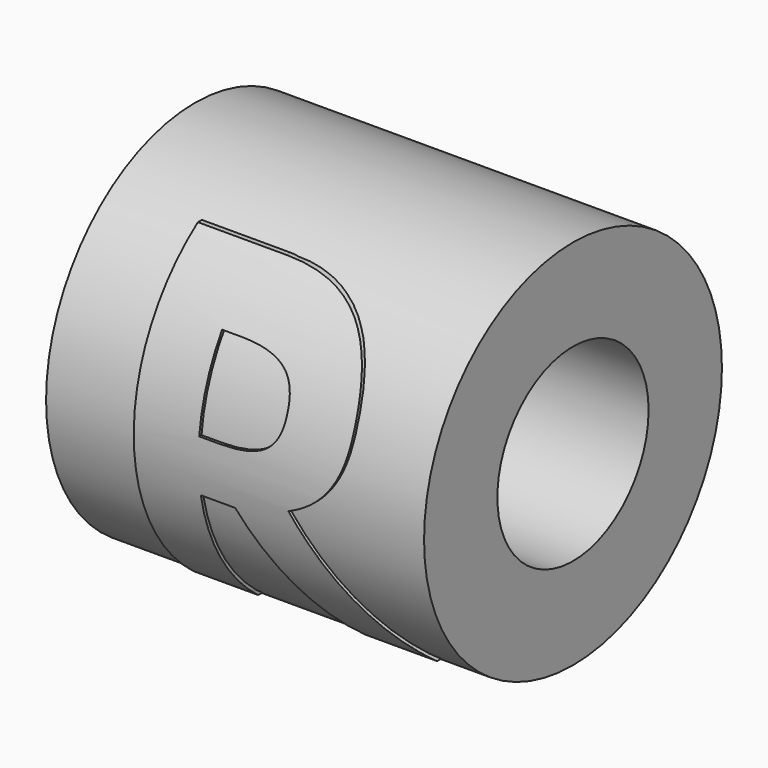
from build123d import *

# Parameters (mm, degrees)
F0_R         = 1
F0_R_2       = 0.985
F0_R_3       = 0.5
F1_DEPTH     = 2
F2_TEXT_SIZE = 2.2604994431
F3_REACH     = 3.0665061896
F4_DEPTH     = 2


# Not quite as in the source:
# - Text() gives the source's letters only with a copy of the font that has no kerning and outlines rounded to 1/6400 em; it was checked with that copy


with BuildPart() as f1:
    # F0 (on Right) → F1 (new body)
    with BuildSketch(Plane.YZ):
        Circle(F0_R)
        Circle(F0_R_2, mode=Mode.SUBTRACT)
        Circle(F0_R_2)
        Circle(F0_R_3, mode=Mode.SUBTRACT)
    extrude(amount=F1_DEPTH)

    f3_end = f1.faces().sort_by_distance((1, -1, 0))[0]
    # F2 (on Front) → F3 (intersect, up to a face of the model that its end follows)
    with BuildSketch(Plane.XZ):
        with Locations((0.2728080435, -0.7963191019)):
            Text('R', F2_TEXT_SIZE, font='Open Sans', font_style=FontStyle.BOLD, text_align=(TextAlign.LEFT, TextAlign.BOTTOM))
    f3_long = extrude(amount=F3_REACH, mode=Mode.PRIVATE)
    add(split(f3_long, bisect_by=f3_end, keep=Keep.BOTTOM, mode=Mode.PRIVATE), mode=Mode.INTERSECT)


with BuildPart() as f4:
    # F0 (on Right) → F4 (new body)
    with BuildSketch(Plane.YZ):
        Circle(F0_R_2)
        Circle(F0_R_3, mode=Mode.SUBTRACT)
    extrude(amount=F4_DEPTH)


solid = Compound([f1.part, f4.part])
